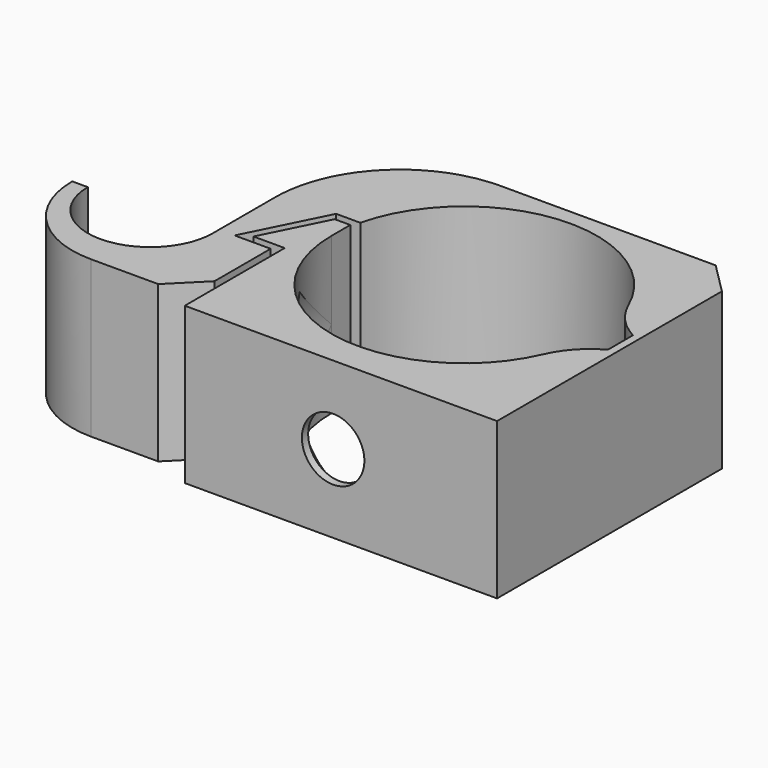
from build123d import *

# Parameters (mm, degrees)
F1_DEPTH    = 5
F4_SIZE     = 2
F5_R        = 5.99999
F6_SIZE     = 4
F7_R        = 10
F8_R        = 8
F9_T1_DEPTH = 22.4376803184
F9_T3_DEPTH = 16.4376803184
F9_T5_DEPTH = 16.4376803184
F10_SIZE    = 2


# Not quite as in the source:
# - a fillet or chamfer that OpenCascade refuses, or shapes differently, is made with other operations: its cross-section is extruded or revolved along the edge and cut away or added
# - a fillet or chamfer is up to 0.001 mm smaller than in the source, because OpenCascade refuses the exact size


with BuildPart() as f1:
    # F0 (on Top) → F1 (new body, symmetric)
    with BuildSketch(Plane.XY):
        with BuildLine():
            ThreePointArc((8.4409715081, -1), (-0.5008703332, -8.4852300446), (-8.5, 0))
            Line((-8.5, 0), (-8.5, 1.5))
            Line((-8.5, 1.5), (-9.5, 1.5))
            Line((-9.5, 1.5), (-11.5, -2.5))
            Line((-11.5, -2.5), (-9.5, -2.5))
            Line((-9.5, -2.5), (-9.5, -10.5))
            Line((-9.5, -10.5), (10.5, -10.5))
            Line((10.5, -10.5), (10.5, 9.5))
            Line((10.5, 9.5), (-13.3090169944, 9.5))
            Line((-13.3090169944, 9.5), (-13.3090169944, -3.5))
            ThreePointArc((-13.3090169944, -3.5), (-17.3090169944, -7.5), (-21.3090169944, -3.5))
            Line((-21.3090169944, -3.5), (-22.3090169944, -3.5))
            Line((-22.3090169944, -3.5), (-22.3090169944, -9.5))
            Line((-22.3090169944, -9.5), (-13.3090169944, -9.5))
            Line((-13.3090169944, -9.5), (-10, -9.5))
            Line((-10, -9.5), (-10, -3))
            Line((-10, -3), (-12.3090169944, -3))
            Line((-12.3090169944, -3), (-9.8090169944, 2))
            Line((-9.8090169944, 2), (-8.2613558209, 2))
            ThreePointArc((-8.2613558209, 2), (0.5080014259, 8.4848060998), (8.4409715081, 1))
            Line((8.4409715081, 1), (10, 1))
            Line((10, 1), (10, -1))
            Line((10, -1), (8.4409715081, -1))
        make_face()
    extrude(amount=F1_DEPTH, both=True)

    # F2 (on Top) → F3 (revolve, cut)
    with BuildSketch(Plane.XY):
        Polygon((0, 0), (-8.5, 0), (-8.5, -3.5), (-2, -10), (-2, -10.5), (0, -10.5), align=None)
    revolve(axis=Axis((0, -4.5, 0), (0, -1, 0)), mode=Mode.SUBTRACT)

    # F4
    f4_edges = [f1.edges().sort_by_distance(p)[0] for p in [
        (-10, -9.5, 0),
    ]]
    chamfer(f4_edges, length=F4_SIZE)

    # F5 (radius 6 in the source; OpenCascade refuses exactly that, so slightly less here)
    f5_edges = [f1.edges().sort_by_distance(p)[0] for p in [
        (-22.309017, -9.5, 0),
    ]]
    fillet(f5_edges, radius=F5_R)

    # F6
    f6_edges = [f1.edges().sort_by_distance(p)[0] for p in [
        (-13.309017, 9.5, 0),
    ]]
    chamfer(f6_edges, length=F6_SIZE)

    # F7
    f7_edges = [f1.edges().sort_by_distance(p)[0] for p in [
        (-9.309017, 9.5, 0),
    ]]
    fillet(f7_edges, radius=F7_R)

    # F8
    f8_edges = [f1.edges().sort_by_distance(p)[0] for p in [
        (-13.309017, 5.5, 0),
    ]]
    fillet(f8_edges, radius=F8_R)

    # F9: fillet of radius 5 on 3 edges, made by hand

    # F9_s2 → F9_t1 (cut)
    with BuildSketch(Plane.XY.offset(-11.2188401592)):
        with BuildLine():
            ThreePointArc((10, 1), (8.693634047, 2.015063424), (7.7900075738, 3.4008501878))
            Line((7.7900075738, 3.4008501878), (7.6983604259, 3.3608401856))
            ThreePointArc((7.6983604259, 3.3608401856), (8.1072760601, 2.1981980996), (8.3416659609, 0.9882352941))
            Line((8.3416659609, 0.9882352941), (8.4409715081, 0.9))
            ThreePointArc((8.4409715081, 0.9), (9.220485754, 0.9), (9.9525527006, 0.911972994))
            Line((9.9525527006, 0.911972994), (10, 1))
        make_face()
    extrude(amount=F9_T1_DEPTH, mode=Mode.SUBTRACT)

    # F9_s4 → F9_t3 (cut)
    with BuildSketch(Plane.XY.offset(-11.2188401592)):
        with BuildLine():
            ThreePointArc((7.7900075738, -3.4008501878), (8.693634047, -2.015063424), (10, -1))
            Line((10, -1), (9.9525527006, -0.911972994))
            ThreePointArc((9.9525527006, -0.911972994), (9.220485754, -0.9), (8.4409715081, -0.9))
            Line((8.4409715081, -0.9), (8.3416659609, -0.9882352941))
            ThreePointArc((8.3416659609, -0.9882352941), (8.1072760601, -2.1981980996), (7.6983604259, -3.3608401856))
            Line((7.6983604259, -3.3608401856), (7.7900075738, -3.4008501878))
        make_face()
    extrude(amount=F9_T3_DEPTH, mode=Mode.SUBTRACT)

    # F9_s6 → F9_t5 (cut)
    with BuildSketch(Plane.XY.offset(-5.2188401592)):
        with BuildLine():
            ThreePointArc((7.7900075738, -3.4008501878), (8.693634047, -2.015063424), (10, -1))
            Line((10, -1), (9.9525527006, -0.911972994))
            ThreePointArc((9.9525527006, -0.911972994), (9.220485754, -0.9), (8.4409715081, -0.9))
            Line((8.4409715081, -0.9), (8.3416659609, -0.9882352941))
            ThreePointArc((8.3416659609, -0.9882352941), (8.1072760601, -2.1981980996), (7.6983604259, -3.3608401856))
            Line((7.6983604259, -3.3608401856), (7.7900075738, -3.4008501878))
        make_face()
    extrude(amount=F9_T5_DEPTH, mode=Mode.SUBTRACT)

    # F10
    f10_edges = [f1.edges().sort_by_distance(p)[0] for p in [
        (10.5, 9.5, 0),
    ]]
    chamfer(f10_edges, length=F10_SIZE)


solid = f1.part
